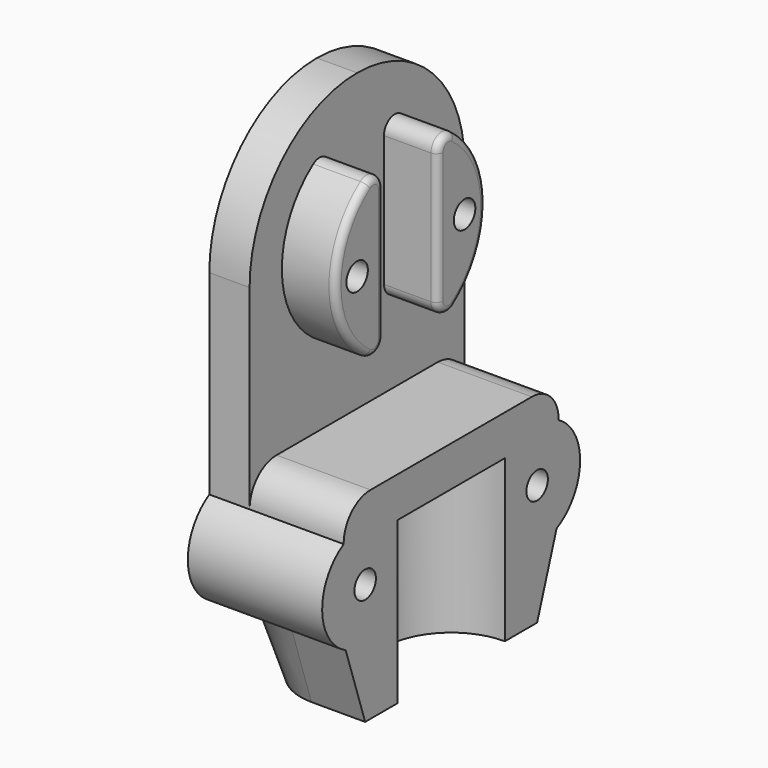
from build123d import *

# Parameters (mm, degrees)
F0_R          = 1
F2_DEPTH      = 7
F3_DEPTH      = 10
F3_DEPTH_BACK = 10
F4_W          = 3
F4_H          = 15
F5_DEPTH      = 10
F5_DEPTH_BACK = 10
F6_R          = 0.5
F7_DEPTH      = 25
F8_R          = 4
F8_R_2        = 2.5
F8_R_3        = 1
F9_DEPTH      = 10
F11_DEPTH     = 12
F12_R         = 2.5
F13_DEPTH     = 2
F14_DEPTH     = 25
F15_R         = 5.99999
F16_T1_DEPTH  = 8.00002
F16_T6_ANGLE  = 90
F16_S7_R      = 4
F16_T8_DEPTH  = 7
F16_T12_ANGLE = 90
F16_S13_R     = 4
F16_T14_DEPTH = 7
F16_T18_DEPTH = 19.5703760639
F16_S19_R     = 4
F16_T20_DEPTH = 12
F16_T24_DEPTH = 19.5703760639
F16_S25_R     = 4
F16_T26_DEPTH = 12
F17_R         = 9.99999
F18_R         = 2.5
F18_R_2       = 1
F19_DEPTH     = 1
F20_R         = 2.5


# Not quite as in the source:
# - a fillet or chamfer that OpenCascade refuses, or shapes differently, is made with other operations: its cross-section is extruded or revolved along the edge and cut away or added
# - a fillet or chamfer is up to 0.001 mm smaller than in the source, because OpenCascade refuses the exact size


with BuildPart() as f2:
    # F0 (on Right) → F2 (new body)
    with BuildSketch(Plane.YZ):
        with BuildLine():
            ThreePointArc((-2.5, 4.8733971724), (-3.0435645354, 5.7631536934), (-4.0833333333, 5.6856300345))
            ThreePointArc((-4.0833333333, 5.6856300345), (-7, 0), (-4.0833333333, -5.6856300345))
            ThreePointArc((-4.0833333333, -5.6856300345), (-3.0435645354, -5.7631536934), (-2.5, -4.8733971724))
            Line((-2.5, -4.8733971724), (-2.5, 0))
            Line((-2.5, 0), (-2.5, 4.8733971724))
        make_face()
        with Locations((-5, 0)):
            Circle(F0_R, mode=Mode.SUBTRACT)
    extrude(amount=-F2_DEPTH)



with BuildPart() as f2b:
    # F0 (on Right) → F2, piece 2 (new body)
    with BuildSketch(Plane.YZ):
        with BuildLine():
            Line((2.5, 4.8733971724), (2.5, 0))
            Line((2.5, 0), (2.5, -4.8733971724))
            ThreePointArc((2.5, -4.8733971724), (3.0435645354, -5.7631536934), (4.0833333333, -5.6856300345))
            ThreePointArc((4.0833333333, -5.6856300345), (7, 0), (4.0833333333, 5.6856300345))
            ThreePointArc((4.0833333333, 5.6856300345), (3.0435645354, 5.7631536934), (2.5, 4.8733971724))
        make_face()
        with Locations((5, 0)):
            Circle(F0_R, mode=Mode.SUBTRACT)
    extrude(amount=-F2_DEPTH)


with BuildPart() as f2_1:
    add(f2.part)

    add(f2b.part)  # F3 merges F2b
    # F1 (on Front) → F3 (join, two sides)
    with BuildSketch(Plane.XZ) as f3_sk:
        Polygon((0, -12), (-7, -12), (-7, 10), (-10, 10), (-10, -27), (0, -27), align=None)
    extrude(amount=F3_DEPTH)
    extrude(f3_sk.sketch, amount=-F3_DEPTH_BACK)

    # F4 (on Front) → F5 (cut, two sides)
    with BuildSketch(Plane.XZ) as f5_sk:
        with Locations((-1.5, 0)):
            Rectangle(F4_W, F4_H)
    extrude(amount=-F5_DEPTH, mode=Mode.SUBTRACT)
    extrude(f5_sk.sketch, amount=F5_DEPTH_BACK, mode=Mode.SUBTRACT)

    # F6
    f6_edges = [f2_1.edges().sort_by_distance(p)[0] for p in [
        (-3, -7, 0),
        (-3, 2.5, 0),
        (-3, -3.043565, 5.763154),
        (-3, -3.043565, -5.763154),
        (-3, -2.5, 0),
        (-3, 7, 0),
        (-3, 3.043565, -5.763154),
        (-3, 3.043565, 5.763154),
    ]]
    fillet(f6_edges, radius=F6_R)

    # F0 (on Right) → F7 (cut)
    with BuildSketch(Plane.YZ):
        with Locations((-8, -18)):
            Circle(F0_R)
        with Locations((8, -18)):
            Circle(F0_R)
    extrude(amount=-F7_DEPTH, mode=Mode.SUBTRACT)

    # F8 (on Right) → F9 (join)
    with BuildSketch(Plane.YZ):
        with Locations((8, -18)):
            Circle(F8_R)
        with Locations((8, -18)):
            Circle(F8_R_2, mode=Mode.SUBTRACT)
        with Locations((-8, -18)):
            Circle(F8_R)
        with Locations((-8, -18)):
            Circle(F8_R_2, mode=Mode.SUBTRACT)
        with Locations((8, -18)):
            Circle(F8_R_2)
        with Locations((8, -18)):
            Circle(F8_R_3, mode=Mode.SUBTRACT)
        with Locations((-8, -18)):
            Circle(F8_R_2)
        with Locations((-8, -18)):
            Circle(F8_R_3, mode=Mode.SUBTRACT)
    extrude(amount=-F9_DEPTH)

    # F10 (on face) → F11 (cut)
    with BuildSketch(Plane(origin=(0, 0, -27), x_dir=(1, 0, 0), z_dir=(0, 0, -1))):
        with BuildLine():
            Line((0, -5), (0, 5))
            ThreePointArc((0, 5), (-5, 0), (0, -5))
        make_face()
    extrude(amount=-F11_DEPTH, mode=Mode.SUBTRACT)

    # F12 (on face) → F13 (cut)
    with BuildSketch(Plane(origin=(-10, 0, 0), x_dir=(0, -1, 0), z_dir=(-1, 0, 0))):
        with Locations((-8, -18)):
            Circle(F12_R)
        with Locations((8, -18)):
            Circle(F12_R)
    extrude(amount=-F13_DEPTH, mode=Mode.SUBTRACT)

    # F0 (on Right) → F14 (cut)
    with BuildSketch(Plane.YZ):
        with Locations((-5, 0)):
            Circle(F0_R)
        with Locations((5, 0)):
            Circle(F0_R)
    extrude(amount=-F14_DEPTH, mode=Mode.SUBTRACT)

    # F15 (radius 6 in the source; OpenCascade refuses exactly that, so slightly less here)
    f15_edges = [f2_1.edges().sort_by_distance(p)[0] for p in [
        (-10, 10, -24.232051),
        (-10, -10, -24.232051),
    ]]
    fillet(f15_edges, radius=F15_R)

    # F16: chamfer of 2 x 6 on 5 edges, made by hand

    # F16_s2 → F16_t1 (cut)
    with BuildSketch(Plane.XZ.offset(-4.00001)):
        Polygon((-10, -21), (-8, -27), (-10, -27), align=None)
    extrude(amount=F16_T1_DEPTH, mode=Mode.SUBTRACT)


with BuildPart() as f16_tool4:
    # F16_s5 → F16_t6 (revolve)
    with BuildSketch(Plane.XZ.offset(-4.00001)):
        Polygon((-8, -27), (-10, -21), (-10, -27), align=None)
    revolve(axis=Axis((-4.00001, 4.00001, -27), (0, 0, -1)), revolution_arc=F16_T6_ANGLE)

    # F16_s7 → F16_t8 (cut, symmetric)
    with BuildSketch(Plane.YZ.offset(-7)):
        with Locations((8, -18)):
            Circle(F16_S7_R)
    extrude(amount=F16_T8_DEPTH, both=True, mode=Mode.SUBTRACT)


with BuildPart() as f2_2:
    add(f2_1.part)

    # F16_t3: cut F16_tool4
    add(f16_tool4.part, mode=Mode.SUBTRACT)


with BuildPart() as f16_tool10:
    # F16_s11 → F16_t12 (revolve)
    with BuildSketch(Plane.XZ.offset(4.00001)):
        Polygon((-8, -27), (-10, -21), (-10, -27), align=None)
    revolve(axis=Axis((-4.00001, -4.00001, -27), (0, 0, 1)), revolution_arc=F16_T12_ANGLE)

    # F16_s13 → F16_t14 (cut, symmetric)
    with BuildSketch(Plane.YZ.offset(-7)):
        with Locations((-8, -18)):
            Circle(F16_S13_R)
    extrude(amount=F16_T14_DEPTH, both=True, mode=Mode.SUBTRACT)


with BuildPart() as f2_3:
    add(f2_2.part)

    # F16_t9: cut F16_tool10
    add(f16_tool10.part, mode=Mode.SUBTRACT)


with BuildPart() as f16_tool16:
    # F16_s17 → F16_t18 (new body)
    with BuildSketch(Plane.YZ.offset(-4.00001)):
        Polygon((-8, -27), (-10, -21), (-10, -27), align=None)
    extrude(amount=F16_T18_DEPTH)

    # F16_s19 → F16_t20 (cut, symmetric)
    with BuildSketch(Plane.YZ.offset(5.8)):
        with Locations((-8, -18)):
            Circle(F16_S19_R)
    extrude(amount=F16_T20_DEPTH, both=True, mode=Mode.SUBTRACT)


with BuildPart() as f2_4:
    add(f2_3.part)

    # F16_t15: cut F16_tool16
    add(f16_tool16.part, mode=Mode.SUBTRACT)


with BuildPart() as f16_tool22:
    # F16_s23 → F16_t24 (new body)
    with BuildSketch(Plane.YZ.offset(-4.00001)):
        Polygon((8, -27), (10, -21), (10, -27), align=None)
    extrude(amount=F16_T24_DEPTH)

    # F16_s25 → F16_t26 (cut, symmetric)
    with BuildSketch(Plane.YZ.offset(5.8)):
        with Locations((8, -18)):
            Circle(F16_S25_R)
    extrude(amount=F16_T26_DEPTH, both=True, mode=Mode.SUBTRACT)


with BuildPart() as f2_5:
    add(f2_4.part)

    # F16_t21: cut F16_tool22
    add(f16_tool22.part, mode=Mode.SUBTRACT)

    # F17 (radius 10 in the source; OpenCascade refuses exactly that, so slightly less here)
    f17_edges = [f2_5.edges().sort_by_distance(p)[0] for p in [
        (-8.5, -10, 10),
        (-8.5, 10, 10),
    ]]
    fillet(f17_edges, radius=F17_R)

    # F18 (on face) → F19 (cut)
    with BuildSketch(Plane(origin=(-10, 0, 0), x_dir=(0, -1, 0), z_dir=(-1, 0, 0))):
        with Locations((-5, 0)):
            Circle(F18_R)
        with Locations((-5, 0)):
            Circle(F18_R_2, mode=Mode.SUBTRACT)
        with Locations((5, 0)):
            Circle(F18_R)
        with Locations((5, 0)):
            Circle(F18_R_2, mode=Mode.SUBTRACT)
    extrude(amount=-F19_DEPTH, mode=Mode.SUBTRACT)

    # F20
    f20_edges = [f2_5.edges().sort_by_distance(p)[0] for p in [
        (-3.5, 10, -12),
        (-3.5, -10, -12),
    ]]
    fillet(f20_edges, radius=F20_R)


solid = f2_5.part
